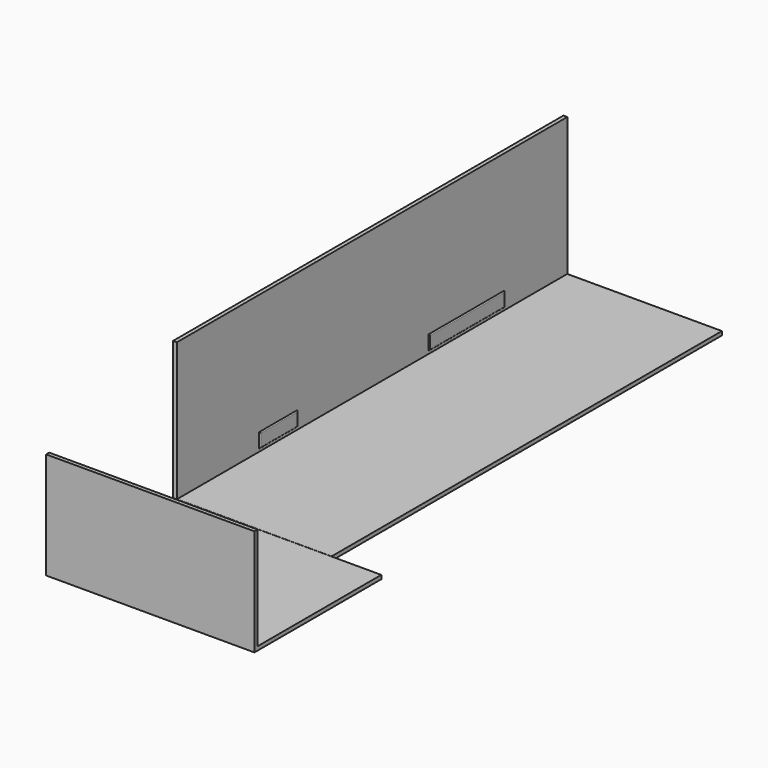
from build123d import *

# Parameters (mm, degrees)
F1_DEPTH = 1199
F2_W     = 233
F2_H     = 70
F2_W_2   = 465
F3_DEPTH = 5
F4_R     = 4.99999
F6_DEPTH = 1024


# Not quite as in the source:
# - a fillet or chamfer is up to 0.001 mm smaller than in the source, because OpenCascade refuses the exact size


with BuildPart() as f1:
    # F0 (on Front) → F1 (new body, symmetric)
    with BuildSketch(Plane.XZ):
        Polygon((380, -339.5), (-380, -339.5), (-380, 339.5), (-398.9999890327, 339.4795854083), (-398.9999890327, -358.4999890327), (380.0204145917, -358.4999890327), align=None)
    extrude(amount=F1_DEPTH, both=True)

    # F2 (on face) → F3 (join)
    with BuildSketch(Plane.YZ.offset(-380)):
        with Locations((-577.5, -289.5)):
            Rectangle(F2_W, F2_H)
        with Locations((578.5, -289.5)):
            Rectangle(F2_W_2, F2_H)
    extrude(amount=F3_DEPTH)

    # F4 (radius 5 in the source; OpenCascade refuses exactly that, so slightly less here)
    f4_edges = [f1.edges().sort_by_distance(p)[0] for p in [
        (-375, -577.5, -254.5),
        (-375, -694, -289.5),
        (-375, -577.5, -324.5),
        (-375, -461, -289.5),
        (-375, 811, -289.5),
        (-375, 578.5, -254.5),
        (-375, 346, -289.5),
        (-375, 578.5, -324.5),
    ]]
    fillet(f4_edges, radius=F4_R)


with BuildPart() as f6:
    # F5 (on face) → F6 (new body)
    with BuildSketch(Plane(origin=(-398.9999890327, 0, 0), x_dir=(0, -1, 0), z_dir=(-1, 0, 0))):
        Polygon((1979, 165.5000109673), (1960, 165.5000109673), (1960, -339.4999890327), (1200, -339.4999890327), (1200, -358.4999890327), (1979, -358.4999890327), align=None)
    extrude(amount=-F6_DEPTH)


solid = Compound([f1.part, f6.part])
